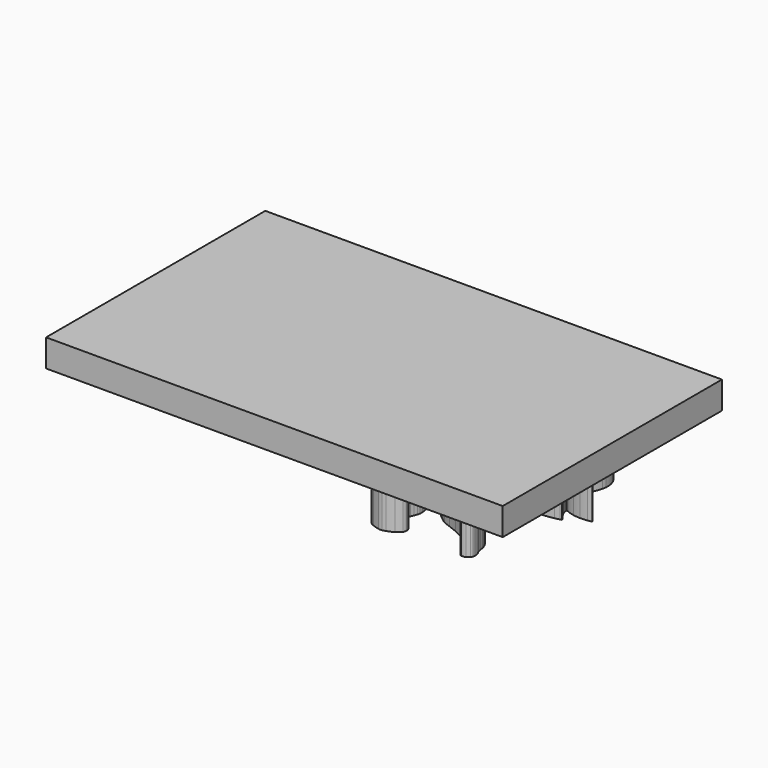
from build123d import *

# Parameters (mm, degrees)
F0_W         = 50
F0_H         = 30
F1_DEPTH     = 3
F3_DEPTH     = 7
F4_TEXT_SIZE = 8.3333333333
F5_DEPTH     = 7


# Not quite as in the source:
# - ends of sketch curves that miss each other by under 0.0002 mm in the source are joined
# - Text() gives the source's letters only with a copy of the font that has no kerning and outlines rounded to 1/6400 em; it was checked with that copy


with BuildPart() as f1:
    # F0 (on Top) → F1 (new body)
    with BuildSketch(Plane.XY):
        Rectangle(F0_W, F0_H)
    extrude(amount=F1_DEPTH)

    # F2 (on face) → F3 (join)
    with BuildSketch(Plane.XY.offset(3)):
        with BuildLine():
            ThreePointArc((22.1029319374, -3.3426466462), (22.1335927234, -3.3306049151), (22.1571887776, -3.307619848))
            ThreePointArc((22.1571887776, -3.307619848), (22.1344498434, -3.2562409626), (22.1018001787, -3.2105148427))
            ThreePointArc((22.1018001787, -3.2105148427), (22.0323939631, -3.1224909159), (21.9593477204, -3.0374633543))
            ThreePointArc((21.9593477204, -3.0374633543), (21.703204298, -2.6741192805), (21.5030609874, -2.2771670052))
            ThreePointArc((21.5030609874, -2.2771670052), (21.463904706, -2.1767883277), (21.4302218121, -2.0744430563))
            ThreePointArc((21.4302218121, -2.0744430563), (21.402616107, -1.9712301339), (21.3892138358, -1.8652330676))
            ThreePointArc((21.3892138358, -1.8652330676), (21.3924565661, -1.8126015358), (21.4128440011, -1.7639710007))
            ThreePointArc((21.4128440011, -1.7639710007), (21.4337557491, -1.748190067), (21.4594309845, -1.742981672))
            ThreePointArc((21.4594309845, -1.742981672), (21.5107043665, -1.7549796998), (21.5600612529, -1.7733324323))
            ThreePointArc((21.5600612529, -1.7733324323), (21.9489169991, -1.9314927468), (22.3564250342, -2.0322928014))
            ThreePointArc((22.3564250342, -2.0322928014), (22.7585600128, -2.0944241547), (23.1647969996, -2.1177560421))
            ThreePointArc((23.1647969996, -2.1177560421), (23.5587988517, -2.1034589577), (23.9509860545, -2.0630723992))
            ThreePointArc((23.9509860545, -2.0630723992), (24.1390155469, -2.0300966659), (24.3227092933, -1.9781438659))
            ThreePointArc((24.3227092933, -1.9781438659), (24.3440205066, -1.9682614631), (24.3640993197, -1.9560684658))
            ThreePointArc((24.3640993197, -1.9560684658), (24.3823476101, -1.9419461804), (24.3894938418, -1.9200059974))
            ThreePointArc((24.3894938418, -1.9200059974), (24.3562440228, -1.8878426607), (24.3120610078, -1.8741348838))
            ThreePointArc((24.3120610078, -1.8741348838), (24.2209460938, -1.8542683499), (24.1285569189, -1.8415858315))
            ThreePointArc((24.1285569189, -1.8415858315), (23.7652342198, -1.7709183165), (23.4064568602, -1.6799454929))
            ThreePointArc((23.4064568602, -1.6799454929), (22.7248477158, -1.4575366039), (22.0667941887, -1.1728926139))
            ThreePointArc((22.0667941887, -1.1728926139), (21.7694202617, -1.0160837141), (21.4794586666, -0.8459585398))
            ThreePointArc((21.4794586666, -0.8459585398), (20.9531272262, -0.4628777243), (20.4811846933, -0.0144962833))
            ThreePointArc((20.4811846933, -0.0144962833), (20.3736737412, 0.0939068753), (20.2636547348, 0.1997637178))
            ThreePointArc((20.2636547348, 0.1997637178), (20.2086041991, 0.25091078), (20.1523350217, 0.3007140251))
            Line((20.1523350217, 0.3007140251), (20.094868, 0.348202))
            ThreePointArc((20.094868, 0.348202), (20.0801541848, 0.3595082308), (20.0641942115, 0.3689744108))
            ThreePointArc((20.0641942115, 0.3689744108), (20.0475263762, 0.3764051613), (20.0293219803, 0.3751270605))
            ThreePointArc((20.0293219803, 0.3751270605), (19.9600511942, 0.3494076822), (19.89527878, 0.3138483392))
            ThreePointArc((19.89527878, 0.3138483392), (19.7709191372, 0.2358938643), (19.6466515879, 0.1577926549))
            ThreePointArc((19.6466515879, 0.1577926549), (19.1323196681, -0.1049678817), (18.5867059713, -0.2944058944))
            Line((18.5867059713, -0.2944058944), (18.066818, -0.447047))
            ThreePointArc((18.066818, -0.447047), (17.5495498471, -0.5359859318), (17.0275689786, -0.5908717027))
            ThreePointArc((17.0275689786, -0.5908717027), (16.7817640364, -0.6018477452), (16.5357229614, -0.5997641021))
            ThreePointArc((16.5357229614, -0.5997641021), (16.0627535258, -0.5467587051), (15.6121118514, -0.3936843195))
            ThreePointArc((15.6121118514, -0.3936843195), (15.5121565594, -0.3438449648), (15.4180749744, -0.2836480357))
            ThreePointArc((15.4180749744, -0.2836480357), (15.3361559268, -0.2114465101), (15.2878162741, -0.113532926))
            ThreePointArc((15.2878162741, -0.113532926), (15.2848405604, -0.0596137865), (15.2951917862, -0.0066139299))
            ThreePointArc((15.2951917862, -0.0066139299), (15.3474223017, 0.0870140055), (15.4128896039, 0.1719153551))
            ThreePointArc((15.4128896039, 0.1719153551), (15.5657152405, 0.3175623213), (15.7453867634, 0.4284084916))
            ThreePointArc((15.7453867634, 0.4284084916), (15.9367202099, 0.5015461272), (16.1335889662, 0.5581171399))
            ThreePointArc((16.1335889662, 0.5581171399), (16.5241597601, 0.6288756157), (16.9172669009, 0.6838218309))
            ThreePointArc((16.9172669009, 0.6838218309), (17.2872368445, 0.7242678102), (17.6575209129, 0.761727897))
            ThreePointArc((17.6575209129, 0.761727897), (18.003915124, 0.8036136097), (18.3495499598, 0.8513622738))
            ThreePointArc((18.3495499598, 0.8513622738), (18.6708573465, 0.9123089639), (18.9866486926, 0.997330991))
            ThreePointArc((18.9866486926, 0.997330991), (19.2746065376, 1.1023873017), (19.5503467529, 1.236267449))
            ThreePointArc((19.5503467529, 1.236267449), (20.0363217427, 1.5430021297), (20.4872480157, 1.899265119))
            ThreePointArc((20.4872480157, 1.899265119), (20.6679326764, 2.0741292052), (20.8285529599, 2.2675860297))
            ThreePointArc((20.8285529599, 2.2675860297), (20.8963137401, 2.3640780678), (20.9526583004, 2.4676518581))
            ThreePointArc((20.9526583004, 2.4676518581), (21.1327044798, 2.8873270351), (21.2638100346, 3.3247687532))
            ThreePointArc((21.2638100346, 3.3247687532), (21.3062971025, 3.5200922172), (21.338611858, 3.7173538822))
            ThreePointArc((21.338611858, 3.7173538822), (21.285468396, 4.4617933569), (20.9979760278, 5.1505330173))
            ThreePointArc((20.9979760278, 5.1505330173), (20.8341304413, 5.3786882133), (20.6412024997, 5.5828424592))
            ThreePointArc((20.6412024997, 5.5828424592), (20.4529640216, 5.7411248861), (20.2556632904, 5.8879564154))
            ThreePointArc((20.2556632904, 5.8879564154), (20.0765420123, 6.0071459752), (19.8898036971, 6.1140074266))
            ThreePointArc((19.8898036971, 6.1140074266), (19.8029006818, 6.1502081132), (19.7129129816, 6.177863928))
            ThreePointArc((19.7129129816, 6.177863928), (19.5462940626, 6.2361909329), (19.3837477898, 6.3050575451))
            ThreePointArc((19.3837477898, 6.3050575451), (19.2454351376, 6.3737729502), (19.1138688924, 6.4546588415))
            ThreePointArc((19.1138688924, 6.4546588415), (19.0108050787, 6.5410718374), (18.9465536711, 6.6592288945))
            ThreePointArc((18.9465536711, 6.6592288945), (18.9169395207, 6.7735071829), (18.9101694206, 6.8913659829))
            ThreePointArc((18.9101694206, 6.8913659829), (18.9184811627, 6.9421310983), (18.9412085813, 6.9882792897))
            ThreePointArc((18.9412085813, 6.9882792897), (18.9593589086, 7.0042267005), (18.9787751476, 7.0186057822))
            ThreePointArc((18.9787751476, 7.0186057822), (19.0021838863, 7.0581293056), (18.997555694, 7.1038308638))
            ThreePointArc((18.997555694, 7.1038308638), (18.9615814572, 7.1278117152), (18.9187770034, 7.1217269938))
            ThreePointArc((18.9187770034, 7.1217269938), (18.8413838243, 7.0930244978), (18.7690869927, 7.0531910112))
            ThreePointArc((18.7690869927, 7.0531910112), (18.2842970335, 6.7385839215), (17.8441801406, 6.364022855))
            Line((17.8441801406, 6.364022855), (17.397998, 6.395694))
            ThreePointArc((17.397998, 6.395694), (17.3103529631, 6.4009592641), (17.2225989991, 6.4038949535))
            ThreePointArc((17.2225989991, 6.4038949535), (16.9920672399, 6.3945578309), (16.7682721326, 6.3384526346))
            ThreePointArc((16.7682721326, 6.3384526346), (16.5938191665, 6.2343978758), (16.4503782753, 6.0905717865))
            ThreePointArc((16.4503782753, 6.0905717865), (16.3966017151, 6.0283346671), (16.3392593586, 5.9693666301))
            ThreePointArc((16.3392593586, 5.9693666301), (16.2812870866, 5.9242270543), (16.2109399831, 5.9030221556))
            ThreePointArc((16.2109399831, 5.9030221556), (16.1330152035, 5.9175870236), (16.061140433, 5.9510300973))
            ThreePointArc((16.061140433, 5.9510300973), (15.9329148518, 6.0022676907), (15.7971719973, 6.0275859684))
            ThreePointArc((15.7971719973, 6.0275859684), (15.7126909251, 6.0145717267), (15.6309458134, 5.9895884833))
            ThreePointArc((15.6309458134, 5.9895884833), (15.4552636216, 5.9196634721), (15.2852713801, 5.8368602882))
            ThreePointArc((15.2852713801, 5.8368602882), (15.1409362293, 5.7543181883), (15.007189314, 5.655537623))
            ThreePointArc((15.007189314, 5.655537623), (14.9197705506, 5.5836607554), (14.8216378843, 5.527284247))
            ThreePointArc((14.8216378843, 5.527284247), (14.6983958368, 5.4969904515), (14.5741337202, 5.5227833859))
            ThreePointArc((14.5741337202, 5.5227833859), (14.4570906064, 5.6162160453), (14.3758933919, 5.7420561708))
            ThreePointArc((14.3758933919, 5.7420561708), (14.2597537925, 5.922939285), (14.1253758851, 6.0907178977))
            ThreePointArc((14.1253758851, 6.0907178977), (14.052523378, 6.178774136), (13.9918877429, 6.2756488618))
            ThreePointArc((13.9918877429, 6.2756488618), (13.9565715528, 6.3943948628), (13.977122648, 6.5165647302))
            ThreePointArc((13.977122648, 6.5165647302), (14.0696746254, 6.6576832211), (14.1907929007, 6.7752021279))
            Line((14.1907929007, 6.7752021279), (14.424397, 6.980828))
            ThreePointArc((14.424397, 6.980828), (14.270314685, 7.2693950633), (14.0967875753, 7.5467047135))
            ThreePointArc((14.0967875753, 7.5467047135), (13.9080082437, 7.8076370193), (13.7130404619, 8.0639783601))
            ThreePointArc((13.7130404619, 8.0639783601), (12.9320566997, 9.063094168), (12.1716875918, 10.0779867007))
            ThreePointArc((12.1716875918, 10.0779867007), (11.9986205712, 10.3196209215), (11.830341284, 10.5646135185))
            ThreePointArc((11.830341284, 10.5646135185), (11.6696754509, 10.8090968239), (11.522150166, 11.0617260912))
            ThreePointArc((11.522150166, 11.0617260912), (11.3903997351, 11.3178257523), (11.2567757293, 11.5729528569))
            ThreePointArc((11.2567757293, 11.5729528569), (11.0010747574, 12.0788202879), (10.793919126, 12.6064293822))
            ThreePointArc((10.793919126, 12.6064293822), (10.7135763429, 12.8689026219), (10.6594022241, 13.1379970338))
            ThreePointArc((10.6594022241, 13.1379970338), (10.6389202457, 13.4074992149), (10.6408091697, 13.6777720402))
            ThreePointArc((10.6408091697, 13.6777720402), (10.6485671228, 13.8105972395), (10.6611547583, 13.9430520274))
            ThreePointArc((10.6611547583, 13.9430520274), (10.6724985861, 14.0080708146), (10.6882235755, 14.0721711195))
            Line((10.6882235755, 14.0721711195), (10.729127, 14.19706))
            ThreePointArc((10.729127, 14.19706), (10.7422439275, 14.2612016768), (10.748636719, 14.326357967))
            ThreePointArc((10.748636719, 14.326357967), (10.7492875956, 14.3589607663), (10.7480104359, 14.39154503))
            ThreePointArc((10.7480104359, 14.39154503), (10.7366969366, 14.4208431644), (10.7084210672, 14.4345129025))
            ThreePointArc((10.7084210672, 14.4345129025), (10.6501175046, 14.4063941926), (10.5967658112, 14.3697402343))
            ThreePointArc((10.5967658112, 14.3697402343), (10.3975648564, 14.2043249689), (10.2003599778, 14.0365350258))
            ThreePointArc((10.2003599778, 14.0365350258), (9.7954861748, 13.7269258234), (9.3691339769, 13.4476330383))
            ThreePointArc((9.3691339769, 13.4476330383), (9.1618467194, 13.3134519806), (8.9553300937, 13.178087858))
            ThreePointArc((8.9553300937, 13.178087858), (8.752286902, 13.044493559), (8.543997929, 12.9192351236))
            ThreePointArc((8.543997929, 12.9192351236), (8.4922109255, 12.88985135), (8.4381049601, 12.8649960977))
            ThreePointArc((8.4381049601, 12.8649960977), (8.4165354678, 12.8460762019), (8.4141984357, 12.8174798236))
            ThreePointArc((8.4141984357, 12.8174798236), (8.4308149291, 12.7929420672), (8.4540191577, 12.7745092759))
            ThreePointArc((8.4540191577, 12.7745092759), (8.553859252, 12.7103891565), (8.6597870306, 12.6569220694))
            ThreePointArc((8.6597870306, 12.6569220694), (8.8734149794, 12.5577061631), (9.0890587594, 12.4629514365))
            ThreePointArc((9.0890587594, 12.4629514365), (9.5076519904, 12.263706548), (9.9058749254, 12.0263498871))
            ThreePointArc((9.9058749254, 12.0263498871), (10.2597394742, 11.7499902359), (10.5810777313, 11.4364037534))
            ThreePointArc((10.5810777313, 11.4364037534), (10.8758121045, 11.1162444535), (11.1546381866, 10.7821391482))
            ThreePointArc((11.1546381866, 10.7821391482), (11.2775516931, 10.6109689174), (11.3872022561, 10.4310141431))
            ThreePointArc((11.3872022561, 10.4310141431), (11.5867607024, 10.0672176183), (11.7652191679, 9.6926190742))
            ThreePointArc((11.7652191679, 9.6926190742), (11.8389524318, 9.5056151586), (11.9059649653, 9.3160989884))
            ThreePointArc((11.9059649653, 9.3160989884), (11.9746417217, 9.1305164923), (12.0468435079, 8.9462768017))
            ThreePointArc((12.0468435079, 8.9462768017), (12.1198954171, 8.7657178025), (12.1853778136, 8.5822779378))
            ThreePointArc((12.1853778136, 8.5822779378), (12.1994845275, 8.5364639036), (12.2126759515, 8.4903779866))
            ThreePointArc((12.2126759515, 8.4903779866), (12.225660459, 8.4444731294), (12.2316767603, 8.3971480395))
            ThreePointArc((12.2316767603, 8.3971480395), (12.231486764, 8.3735887216), (12.2208690488, 8.3525569591))
            ThreePointArc((12.2208690488, 8.3525569591), (12.1566458655, 8.282887717), (12.0838465272, 8.22223565))
            ThreePointArc((12.0838465272, 8.22223565), (11.9327404211, 8.1098500489), (11.7938480882, 7.982678913))
            ThreePointArc((11.7938480882, 7.982678913), (11.5437503461, 7.708873342), (11.3135673737, 7.418125725))
            ThreePointArc((11.3135673737, 7.418125725), (11.1103635725, 7.1218307201), (10.9154264585, 6.8200327128))
            ThreePointArc((10.9154264585, 6.8200327128), (10.7510165266, 6.5134310742), (10.6270360062, 6.1883709981))
            ThreePointArc((10.6270360062, 6.1883709981), (10.5257897909, 5.8667793922), (10.4420216464, 5.5401988526))
            ThreePointArc((10.4420216464, 5.5401988526), (10.3876460738, 5.2181757102), (10.3601916416, 4.8927500153))
            ThreePointArc((10.3601916416, 4.8927500153), (10.3594501629, 4.5764341786), (10.3920034129, 4.2617970649))
            ThreePointArc((10.3920034129, 4.2617970649), (10.4614961842, 3.9634002287), (10.5672791595, 3.6758590701))
            ThreePointArc((10.5672791595, 3.6758590701), (10.6310601771, 3.5418787515), (10.710987144, 3.4168571053))
            ThreePointArc((10.710987144, 3.4168571053), (10.9024251941, 3.1959938332), (11.1098078214, 2.9900288913))
            ThreePointArc((11.1098078214, 2.9900288913), (11.3208907035, 2.8012476911), (11.5216950153, 2.6015680146))
            ThreePointArc((11.5216950153, 2.6015680146), (11.5666479202, 2.5497879326), (11.6078860573, 2.4950033405))
            ThreePointArc((11.6078860573, 2.4950033405), (11.616687903, 2.4299573958), (11.5701631112, 2.3836546665))
            ThreePointArc((11.5701631112, 2.3836546665), (11.5062809929, 2.3624235629), (11.4505536544, 2.324659273))
            ThreePointArc((11.4505536544, 2.324659273), (11.2583689528, 2.138437253), (11.1037236974, 1.9200375973))
            ThreePointArc((11.1037236974, 1.9200375973), (11.0182593854, 1.6756807446), (10.9961275647, 1.4177569827))
            ThreePointArc((10.9961275647, 1.4177569827), (11.0203836963, 1.1675862877), (11.0732531163, 0.9218657558))
            ThreePointArc((11.0732531163, 0.9218657558), (11.1063950755, 0.8046533925), (11.1380252732, 0.6870240716))
            ThreePointArc((11.1380252732, 0.6870240716), (11.1487849133, 0.6281808958), (11.1454363082, 0.5684559457))
            ThreePointArc((11.1454363082, 0.5684559457), (11.1144252493, 0.5182446639), (11.0684700498, 0.4812179106))
            ThreePointArc((11.0684700498, 0.4812179106), (10.9750625739, 0.4090299996), (10.8816996322, 0.336784475))
            ThreePointArc((10.8816996322, 0.336784475), (10.7899717727, 0.2655948746), (10.7090264291, 0.1823504825))
            ThreePointArc((10.7090264291, 0.1823504825), (10.4603960458, -0.2015259075), (10.2534657549, -0.6093958915))
            ThreePointArc((10.2534657549, -0.6093958915), (10.1273187087, -0.9016381072), (10.0222100301, -1.2020900093))
            ThreePointArc((10.0222100301, -1.2020900093), (9.9711519363, -1.4000209254), (9.9389189497, -1.6018738826))
            ThreePointArc((9.9389189497, -1.6018738826), (9.9001298348, -1.996162263), (9.8915441711, -2.3922609972))
            ThreePointArc((9.8915441711, -2.3922609972), (9.9191848661, -2.7625355649), (9.993916869, -3.1262420358))
            ThreePointArc((9.993916869, -3.1262420358), (10.0841389229, -3.4625882584), (10.1878686419, -3.7950171197))
            Line((10.1878686419, -3.7950171197), (10.309094, -4.097906))
            ThreePointArc((10.309094, -4.097906), (10.3182262061, -4.176007141), (10.2987016765, -4.2521778498))
            ThreePointArc((10.2987016765, -4.2521778498), (10.2133345979, -4.3822246874), (10.1131948905, -4.5012698962))
            ThreePointArc((10.1131948905, -4.5012698962), (10.0209350925, -4.6205205207), (9.9392221389, -4.7472310814))
            ThreePointArc((9.9392221389, -4.7472310814), (9.6446140887, -5.251910171), (9.3796218633, -5.7727489353))
            ThreePointArc((9.3796218633, -5.7727489353), (9.2717939129, -6.0045673723), (9.1722547425, -6.2400638965))
            ThreePointArc((9.1722547425, -6.2400638965), (9.0968111802, -6.4675270222), (9.0337928277, -6.698740958))
            ThreePointArc((9.0337928277, -6.698740958), (8.8116512482, -7.5697677788), (8.6121180842, -8.446250018))
            ThreePointArc((8.6121180842, -8.446250018), (8.5920281211, -8.6134799477), (8.5923493112, -8.7819119805))
            ThreePointArc((8.5923493112, -8.7819119805), (8.6215461038, -9.0964794132), (8.6799835021, -9.406947118))
            ThreePointArc((8.6799835021, -9.406947118), (8.7156970839, -9.5405012217), (8.7585585164, -9.6719358161))
            ThreePointArc((8.7585585164, -9.6719358161), (8.805326955, -9.7928104065), (8.8525577001, -9.913504118))
            ThreePointArc((8.8525577001, -9.913504118), (8.8915856058, -10.0285765785), (8.9254503074, -10.1452729182))
            ThreePointArc((8.9254503074, -10.1452729182), (8.9929007224, -10.3628025227), (9.0851815202, -10.571016247))
            ThreePointArc((9.0851815202, -10.571016247), (9.2667968292, -10.9259197148), (9.4705272994, -11.2686058089))
            ThreePointArc((9.4705272994, -11.2686058089), (9.6369276658, -11.5170156437), (9.8162128747, -11.7562913078))
            ThreePointArc((9.8162128747, -11.7562913078), (9.9647352583, -11.9242901884), (10.1293113061, -12.0765966341))
            ThreePointArc((10.1293113061, -12.0765966341), (10.2599361795, -12.1825650611), (10.3956297456, -12.2819603659))
            ThreePointArc((10.3956297456, -12.2819603659), (10.7964657402, -12.5884679343), (11.1815011151, -12.9146018708))
            ThreePointArc((11.1815011151, -12.9146018708), (11.0999957347, -13.0019557206), (11.0137155759, -13.0845966361))
            ThreePointArc((11.0137155759, -13.0845966361), (10.8286614003, -13.2109608974), (10.6344126766, -13.3226763838))
            ThreePointArc((10.6344126766, -13.3226763838), (10.460818169, -13.4140610613), (10.2856393393, -13.5023706882))
            ThreePointArc((10.2856393393, -13.5023706882), (10.1343691876, -13.5835097824), (9.9847020557, -13.667569097))
            ThreePointArc((9.9847020557, -13.667569097), (9.9212034675, -13.7076512286), (9.8603123588, -13.751593466))
            ThreePointArc((9.8603123588, -13.751593466), (9.8082788438, -13.798302663), (9.7723502425, -13.8582890996))
            ThreePointArc((9.7723502425, -13.8582890996), (9.7751819612, -13.8909215619), (9.7922001398, -13.9189088627))
            ThreePointArc((9.7922001398, -13.9189088627), (9.9724493004, -14.098946389), (10.2000738627, -14.2133594341))
            ThreePointArc((10.2000738627, -14.2133594341), (10.5643022818, -14.3337939058), (10.9344281228, -14.4346584969))
            ThreePointArc((10.9344281228, -14.4346584969), (11.1241992017, -14.4604389571), (11.3154450664, -14.450303449))
            ThreePointArc((11.3154450664, -14.450303449), (11.5032870486, -14.4118148566), (11.6859316191, -14.3534459969))
            ThreePointArc((11.6859316191, -14.3534459969), (12.0724332494, -14.2059129649), (12.439371807, -14.0148486765))
            ThreePointArc((12.439371807, -14.0148486765), (12.6986424157, -13.8187595885), (12.9171624868, -13.5780913656))
            ThreePointArc((12.9171624868, -13.5780913656), (13.0051916036, -13.4277018147), (13.0458090983, -13.2582429204))
            ThreePointArc((13.0458090983, -13.2582429204), (13.0390004825, -13.1233772484), (13.0036138397, -12.9930586719))
            ThreePointArc((13.0036138397, -12.9930586719), (12.876573363, -12.7514137309), (12.7083484246, -12.5363976013))
            ThreePointArc((12.7083484246, -12.5363976013), (12.4266710444, -12.249813628), (12.1233380339, -11.9862579577))
            ThreePointArc((12.1233380339, -11.9862579577), (11.9423535894, -11.8090522679), (11.7935047614, -11.6041101444))
            ThreePointArc((11.7935047614, -11.6041101444), (11.6879835404, -11.3901598249), (11.6246509205, -11.1601631897))
            ThreePointArc((11.6246509205, -11.1601631897), (11.6208527253, -11.0518708464), (11.6394906578, -10.9451269028))
            ThreePointArc((11.6394906578, -10.9451269028), (11.6927560741, -10.7794251015), (11.7592413331, -10.6185711537))
            ThreePointArc((11.7592413331, -10.6185711537), (11.8313472203, -10.4449786699), (11.8937250204, -10.2676580066))
            ThreePointArc((11.8937250204, -10.2676580066), (11.9251886808, -10.1534739576), (11.9483854538, -10.0373280738))
            ThreePointArc((11.9483854538, -10.0373280738), (11.9653165732, -9.8619021654), (11.9622944391, -9.6856870415))
            ThreePointArc((11.9622944391, -9.6856870415), (11.9387511421, -9.46837048), (11.9022346538, -9.2528540694))
            ThreePointArc((11.9022346538, -9.2528540694), (11.8706980303, -9.0722699061), (11.8447887544, -8.8907929042))
            ThreePointArc((11.8447887544, -8.8907929042), (11.834146078, -8.8027481062), (11.8370200808, -8.7141090088))
            ThreePointArc((11.8370200808, -8.7141090088), (11.8935443704, -8.6695449594), (11.9554121266, -8.6327572486))
            ThreePointArc((11.9554121266, -8.6327572486), (12.0773164823, -8.5644157455), (12.2012871537, -8.499898307))
            ThreePointArc((12.2012871537, -8.499898307), (12.331324747, -8.4310901488), (12.45836381, -8.3568916898))
            ThreePointArc((12.45836381, -8.3568916898), (12.5341748628, -8.3083441166), (12.6036888729, -8.2511428631))
            ThreePointArc((12.6036888729, -8.2511428631), (12.6596500229, -8.2001135723), (12.729942941, -8.1719257124))
            ThreePointArc((12.729942941, -8.1719257124), (12.7789062563, -8.1944434297), (12.8194004371, -8.2300056278))
            ThreePointArc((12.8194004371, -8.2300056278), (13.05797464, -8.5084966218), (13.2604489964, -8.8142400021))
            ThreePointArc((13.2604489964, -8.8142400021), (13.362115376, -8.9502159867), (13.4782057398, -9.0741052724))
            ThreePointArc((13.4782057398, -9.0741052724), (13.7542552408, -9.3336136986), (14.0446958281, -9.5769082176))
            ThreePointArc((14.0446958281, -9.5769082176), (14.3177848657, -9.7831484959), (14.6071893261, -9.9657894318))
            ThreePointArc((14.6071893261, -9.9657894318), (15.0116436126, -10.1438131154), (15.4259908586, -10.2974104194))
            ThreePointArc((15.4259908586, -10.2974104194), (15.9090916555, -10.4813045224), (16.3848548638, -10.6834253045))
            ThreePointArc((16.3848548638, -10.6834253045), (16.8874441912, -10.9120916794), (17.3821888414, -11.1572693071))
            ThreePointArc((17.3821888414, -11.1572693071), (17.5442634095, -11.2585276432), (17.6984184057, -11.3714774872))
            ThreePointArc((17.6984184057, -11.3714774872), (18.0086402702, -11.6211146894), (18.3078357902, -11.8838662288))
            ThreePointArc((18.3078357902, -11.8838662288), (18.5379065678, -12.1025597511), (18.7489267302, -12.3396882206))
            ThreePointArc((18.7489267302, -12.3396882206), (18.9732644184, -12.6701371229), (19.1766022708, -13.013906851))
            ThreePointArc((19.1766022708, -13.013906851), (19.3103625183, -13.2766318398), (19.4125332482, -13.5531772288))
            ThreePointArc((19.4125332482, -13.5531772288), (19.4494433354, -13.706434972), (19.4874442407, -13.8594259393))
            ThreePointArc((19.4874442407, -13.8594259393), (19.5181955982, -13.8924642025), (19.560962961, -13.9068915021))
            ThreePointArc((19.560962961, -13.9068915021), (19.8107886547, -13.9139736403), (20.0522500402, -13.8494800937))
            ThreePointArc((20.0522500402, -13.8494800937), (20.2104551177, -13.7347743972), (20.3497669475, -13.5977399541))
            ThreePointArc((20.3497669475, -13.5977399541), (20.4223218487, -13.5081302529), (20.4772099173, -13.4067329647))
            ThreePointArc((20.4772099173, -13.4067329647), (20.5026701862, -13.2935602318), (20.5071896431, -13.1776469664))
            ThreePointArc((20.5071896431, -13.1776469664), (20.4581450985, -12.8075249047), (20.2973917776, -12.4705471528))
            ThreePointArc((20.2973917776, -12.4705471528), (20.2498072477, -12.3766805008), (20.2181147423, -12.2763270588))
            ThreePointArc((20.2181147423, -12.2763270588), (20.1838387435, -12.1244817166), (20.1606878552, -11.9705470164))
            ThreePointArc((20.1606878552, -11.9705470164), (20.1394146485, -11.8160069724), (20.1112510014, -11.6625729997))
            ThreePointArc((20.1112510014, -11.6625729997), (20.0878658837, -11.561186837), (20.060132387, -11.4609028839))
            ThreePointArc((20.060132387, -11.4609028839), (19.9654686081, -11.2133297397), (19.8278549824, -10.986799013))
            ThreePointArc((19.8278549824, -10.986799013), (19.7361760403, -10.8908032349), (19.6316579579, -10.8089730626))
            ThreePointArc((19.6316579579, -10.8089730626), (19.4207918921, -10.6793443471), (19.196816126, -10.5739736883))
            ThreePointArc((19.196816126, -10.5739736883), (18.9956363633, -10.5046625647), (18.7853850005, -10.4719259929))
            ThreePointArc((18.7853850005, -10.4719259929), (18.7024144638, -10.4661452902), (18.6210942466, -10.4486941497))
            ThreePointArc((18.6210942466, -10.4486941497), (18.5199889215, -10.4073711756), (18.4318066972, -10.3429213233))
            ThreePointArc((18.4318066972, -10.3429213233), (18.3782966808, -10.2705867277), (18.3571888287, -10.1831220063))
            ThreePointArc((18.3571888287, -10.1831220063), (18.334592353, -10.0959730703), (18.2972319146, -10.0140600484))
            ThreePointArc((18.2972319146, -10.0140600484), (18.1853160649, -9.8070100342), (18.061033615, -9.6071382559))
            ThreePointArc((18.061033615, -9.6071382559), (17.9382874697, -9.4301868694), (17.8001961007, -9.2649319078))
            ThreePointArc((17.8001961007, -9.2649319078), (17.7290501446, -9.2010468683), (17.6530404201, -9.1430334015))
            ThreePointArc((17.6530404201, -9.1430334015), (17.247279623, -8.9026481901), (16.8173336458, -8.7088099189))
            ThreePointArc((16.8173336458, -8.7088099189), (16.3641848824, -8.5483886492), (15.8955619702, -8.4412841771))
            ThreePointArc((15.8955619702, -8.4412841771), (15.8049944661, -8.4269382502), (15.7159648361, -8.4049835611))
            ThreePointArc((15.7159648361, -8.4049835611), (15.6734644858, -8.388723333), (15.6343322167, -8.3654996969))
            ThreePointArc((15.6343322167, -8.3654996969), (15.6002086182, -8.3260215909), (15.5871317953, -8.2755050048))
            ThreePointArc((15.5871317953, -8.2755050048), (15.5953692212, -8.2035903022), (15.6176636315, -8.1347242764))
            ThreePointArc((15.6176636315, -8.1347242764), (15.6438204734, -8.0335650834), (15.6469227872, -7.9291250175))
            ThreePointArc((15.6469227872, -7.9291250175), (15.6237921725, -7.7471582747), (15.5872907858, -7.56739581))
            ThreePointArc((15.5872907858, -7.56739581), (15.4984100142, -7.1859407406), (15.3885038557, -6.8100040466))
            ThreePointArc((15.3885038557, -6.8100040466), (15.3023430115, -6.5845402521), (15.1838937957, -6.3742371359))
            ThreePointArc((15.1838937957, -6.3742371359), (15.1361153256, -6.30743641), (15.0940785918, -6.2368812206))
            ThreePointArc((15.0940785918, -6.2368812206), (15.0677323299, -6.150981423), (15.0775853429, -6.0616741112))
            ThreePointArc((15.0775853429, -6.0616741112), (15.1357112934, -5.9246620957), (15.2084089807, -5.7947929878))
            ThreePointArc((15.2084089807, -5.7947929878), (15.3592939199, -5.4976582221), (15.4704077747, -5.1834782186))
            ThreePointArc((15.4704077747, -5.1834782186), (15.5440489759, -4.8167485136), (15.5793746477, -4.4443699849))
            ThreePointArc((15.5793746477, -4.4443699849), (15.5884382289, -3.9132783027), (15.5354891228, -3.3847549804))
            ThreePointArc((15.5354891228, -3.3847549804), (15.4936475879, -3.1172250803), (15.4627373792, -2.8482129642))
            ThreePointArc((15.4627373792, -2.8482129642), (15.4626025731, -2.813715273), (15.4746326694, -2.7813828035))
            ThreePointArc((15.4746326694, -2.7813828035), (15.4945059498, -2.7724176588), (15.5163020126, -2.77192593))
            ThreePointArc((15.5163020126, -2.77192593), (15.6214591175, -2.8205854806), (15.7206082174, -2.8805456816))
            ThreePointArc((15.7206082174, -2.8805456816), (15.9261318029, -3.0088900206), (16.1288013299, -3.1416969986))
            ThreePointArc((16.1288013299, -3.1416969986), (16.3233107188, -3.2698204627), (16.5210358638, -3.3929232252))
            ThreePointArc((16.5210358638, -3.3929232252), (16.767426247, -3.5277579931), (17.0246719584, -3.6405111074))
            ThreePointArc((17.0246719584, -3.6405111074), (17.3674209778, -3.7596364844), (17.714857054, -3.8643058061))
            ThreePointArc((17.714857054, -3.8643058061), (18.124146591, -3.9675160859), (18.539430996, -4.0430750271))
            ThreePointArc((18.539430996, -4.0430750271), (18.6888440004, -4.0616169764), (18.8391309746, -4.070665893))
            ThreePointArc((18.8391309746, -4.070665893), (18.8824265032, -4.0696944815), (18.925348995, -4.0639409736))
            ThreePointArc((18.925348995, -4.0639409736), (18.9443912342, -4.0580638751), (18.9556283754, -4.0416058319))
            ThreePointArc((18.9556283754, -4.0416058319), (18.9008433018, -3.9153983124), (18.8308856353, -3.7969255697))
            ThreePointArc((18.8308856353, -3.7969255697), (18.7555962016, -3.6379481544), (18.7131368124, -3.4672450273))
            ThreePointArc((18.7131368124, -3.4672450273), (18.7074539971, -3.3978821905), (18.7123177245, -3.3284571064))
            ThreePointArc((18.7123177245, -3.3284571064), (18.7256145211, -3.2835843457), (18.75577744, -3.247799562))
            ThreePointArc((18.75577744, -3.247799562), (18.7896800609, -3.2417022684), (18.8235540999, -3.2479587369))
            ThreePointArc((18.8235540999, -3.2479587369), (18.8725203526, -3.2656642711), (18.918276912, -3.2905141364))
            ThreePointArc((18.918276912, -3.2905141364), (19.1962621459, -3.4161580047), (19.4821888874, -3.5224973376))
            ThreePointArc((19.4821888874, -3.5224973376), (19.7050025879, -3.5989256241), (19.9341800307, -3.6533768358))
            ThreePointArc((19.9341800307, -3.6533768358), (20.1646215373, -3.6662441897), (20.3951859899, -3.6558088953))
            ThreePointArc((20.3951859899, -3.6558088953), (20.9360802002, -3.5930186009), (21.47234225, -3.4985082092))
            ThreePointArc((21.47234225, -3.4985082092), (21.7147904484, -3.4478178181), (21.9554339178, -3.3891546855))
            ThreePointArc((21.9554339178, -3.3891546855), (22.0297873933, -3.3678177989), (22.1029319374, -3.3426466462))
        make_face()
        with BuildLine():
            Line((13.485828, 5.590677), (13.714217, 5.793773))
            Line((13.714217, 5.793773), (13.97773, 5.530261))
            Line((13.97773, 5.530261), (13.891151, 5.289493))
            ThreePointArc((13.891151, 5.289493), (13.8515537858, 5.1591602724), (13.8296609337, 5.0247160063))
            ThreePointArc((13.8296609337, 5.0247160063), (13.8260878869, 4.8589352316), (13.8375849407, 4.6935149932))
            ThreePointArc((13.8375849407, 4.6935149932), (13.8527333536, 4.4965919451), (13.8488625875, 4.299125028))
            ThreePointArc((13.8488625875, 4.299125028), (13.8237719235, 4.1900740913), (13.7617143807, 4.0969586318))
            ThreePointArc((13.7617143807, 4.0969586318), (13.7003064259, 4.0497258317), (13.6320507818, 4.0130785003))
            ThreePointArc((13.6320507818, 4.0130785003), (13.5442136596, 3.9715580175), (13.4537069091, 3.9362332592))
            ThreePointArc((13.4537069091, 3.9362332592), (13.4225762534, 3.9307372867), (13.3971511573, 3.9495225074))
            ThreePointArc((13.3971511573, 3.9495225074), (13.371709512, 3.9844022855), (13.3478438777, 4.0203789227))
            ThreePointArc((13.3478438777, 4.0203789227), (13.3190528785, 4.0702447285), (13.2918115037, 4.1209742606))
            ThreePointArc((13.2918115037, 4.1209742606), (13.1936085748, 4.3292709784), (13.1106249307, 4.5440849761))
            ThreePointArc((13.1106249307, 4.5440849761), (13.062859966, 4.6899070044), (13.0262688988, 4.8389259792))
            ThreePointArc((13.0262688988, 4.8389259792), (13.0275938924, 4.9264467559), (13.0462502475, 5.0119662449))
            ThreePointArc((13.0462502475, 5.0119662449), (13.0843852339, 5.1046327782), (13.1319157762, 5.1928495282))
            ThreePointArc((13.1319157762, 5.1928495282), (13.292873274, 5.4059957845), (13.485828, 5.590677))
        make_face(mode=Mode.SUBTRACT)
        with BuildLine():
            ThreePointArc((12.7886201419, 6.242790003), (12.7663837039, 6.1082620132), (12.6970472875, 5.9908537487))
            ThreePointArc((12.6970472875, 5.9908537487), (12.6768301537, 5.9673549791), (12.6535978679, 5.9468321719))
            ThreePointArc((12.6535978679, 5.9468321719), (12.6307041792, 5.9370150239), (12.6057988178, 5.9365369619))
            ThreePointArc((12.6057988178, 5.9365369619), (12.4981624338, 5.9762134349), (12.3969948106, 6.0302956978))
            Line((12.3969948106, 6.0302956978), (12.211801, 6.128098))
            Line((12.211801, 6.128098), (12.334006, 6.390586))
            ThreePointArc((12.334006, 6.390586), (12.4043772143, 6.5496732045), (12.4567004972, 6.7155741284))
            ThreePointArc((12.4567004972, 6.7155741284), (12.4590121193, 6.7470812397), (12.4747453473, 6.7744766794))
            ThreePointArc((12.4747453473, 6.7744766794), (12.5006061586, 6.776766771), (12.5231260501, 6.7638480463))
            ThreePointArc((12.5231260501, 6.7638480463), (12.6137246338, 6.6653519751), (12.6853006728, 6.5522748319))
            ThreePointArc((12.6853006728, 6.5522748319), (12.756653276, 6.4041067508), (12.7886201419, 6.242790003))
        make_face(mode=Mode.SUBTRACT)
    extrude(amount=-F3_DEPTH)

    # F4 (on face) → F5 (join)
    with BuildSketch(Plane.XY.offset(3)):
        with Locations((-19, 1.630280095)):
            Text('Sabine', F4_TEXT_SIZE, font='Open Sans', font_style=FontStyle.BOLD, text_align=(TextAlign.LEFT, TextAlign.BOTTOM))
        with Locations((-18.2073319873, -8.2816741839)):
            Text('Dirk', F4_TEXT_SIZE, font='Open Sans', font_style=FontStyle.BOLD, text_align=(TextAlign.LEFT, TextAlign.BOTTOM))
    extrude(amount=-F5_DEPTH)


solid = f1.part
